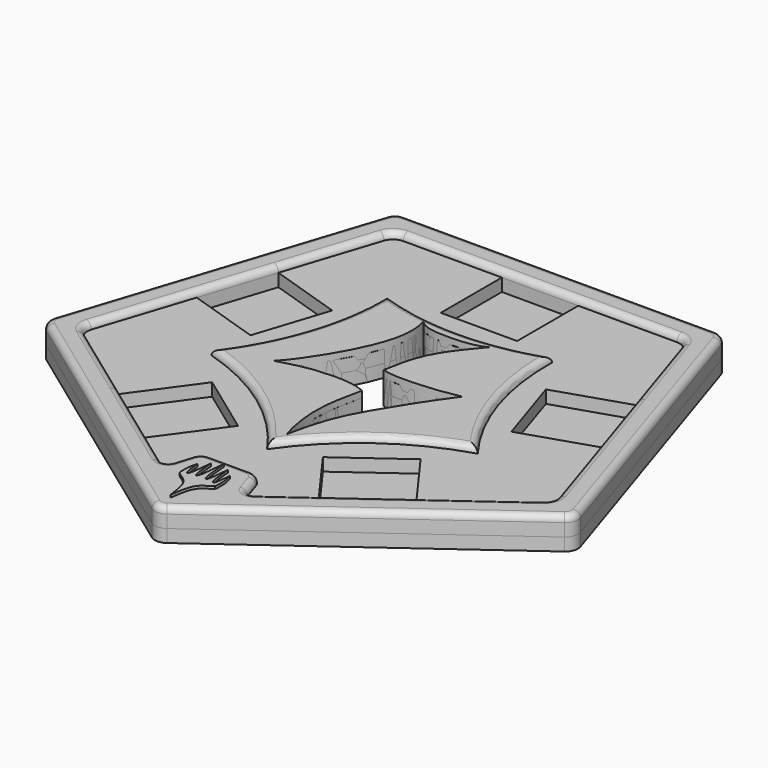
from build123d import *

# Parameters (mm, degrees)
F4_DEPTH      = 2
F5_DEPTH      = 5
F6_DEPTH      = 2
F8_DEPTH      = 5
F9_DEPTH      = 5.001
F10_DEPTH     = 5.4
F11_T2_ANGLE  = 45.9808997244
F11_T4_ANGLE  = 45.9808997244
F11_T6_ANGLE  = 45.9808997244
F11_T8_ANGLE  = 45.9808997244
F11_T10_ANGLE = 45.9808997244
F12_R         = 2
F12_2_R       = 2
F13_R         = 2
F14_R         = 1
F15_R         = 1
F16_R         = 1


# Not quite as in the source:
# - a fillet or chamfer that OpenCascade refuses, or shapes differently, is made with other operations: its cross-section is extruded or revolved along the edge and cut away or added


with BuildPart() as f4:
    # F2 (on Top) → F4 (new body)
    with BuildSketch(Plane.XY):
        Polygon((0, -44), (41.846486717, -13.5967477525), (25.8625511009, 35.5967477525), (-25.8625511009, 35.5967477525), (-41.846486717, -13.5967477525), align=None)
        Polygon((-6.3112691246, -34.4703226653), (-13.7180003831, -29.0890174125), (-23.4262043156, -22.035594385), (-37.1442046986, -12.0688837075), (-31.90439481, 4.0575929247), (-28.1961908775, 15.4702711203), (-22.9563809888, 31.5967477525), (-6, 31.5967477525), (6, 31.5967477525), (22.9563809888, 31.5967477525), (28.1961908775, 15.4702711203), (31.90439481, 4.0575929247), (37.1442046986, -12.0688837075), (23.4262043156, -22.035594385), (13.7180003831, -29.0890174125), (6.3112691246, -34.4703226653), (4.5704734512, -29.0890174125), (-4.6459520236, -29.0890174125), align=None, mode=Mode.SUBTRACT)
        Polygon((-23.4262043156, -22.035594385), (-13.7180003831, -29.0890174125), (-6.3112691246, -34.4703226653), (-4.6459520236, -29.0890174125), (4.5704734512, -29.0890174125), (6.3112691246, -34.4703226653), (13.7180003831, -29.0890174125), (23.4262043156, -22.035594385), (37.1442046986, -12.0688837075), (31.90439481, 4.0575929247), (28.1961908775, 15.4702711203), (22.9563809888, 31.5967477525), (6, 31.5967477525), (-6, 31.5967477525), (-22.9563809888, 31.5967477525), (-28.1961908775, 15.4702711203), (-31.90439481, 4.0575929247), (-37.1442046986, -12.0688837075), align=None)
    extrude(amount=F4_DEPTH)


with BuildPart() as f4b:
    # F0 (on Top) → F4, piece 2 (new body)
    with BuildSketch(Plane.XY):
        Polygon((-16.783512682, 11.7620671878), (-20.4917166145, 0.3493889922), (-31.90439481, 4.0575929247), (-37.1442046986, -12.0688837075), (-23.4262043156, -22.035594385), (-16.3727812881, -12.3273904525), (-6.6645773556, -19.38081348), (-13.7180003831, -29.0890174125), (0, -39.05572809), (13.7180003831, -29.0890174125), (6.6645773556, -19.38081348), (16.3727812881, -12.3273904525), (23.4262043156, -22.035594385), (37.1442046986, -12.0688837075), (31.90439481, 4.0575929247), (20.4917166145, 0.3493889922), (16.783512682, 11.7620671878), (28.1961908775, 15.4702711203), (22.9563809888, 31.5967477525), (6, 31.5967477525), (6, 19.5967477525), (-6, 19.5967477525), (-6, 31.5967477525), (-22.9563809888, 31.5967477525), (-28.1961908775, 15.4702711203), align=None)
        with BuildLine():
            ThreePointArc((0, -22), (-9.1675383126, -12.6180339887), (-20.9232433585, -6.7983738762))
            ThreePointArc((-20.9232433585, -6.7983738762), (-14.833388583, 4.8196601125), (-12.9312755504, 17.7983738762))
            ThreePointArc((-12.9312755504, 17.7983738762), (0, 15.5967477525), (12.9312755504, 17.7983738762))
            ThreePointArc((12.9312755504, 17.7983738762), (14.833388583, 4.8196601125), (20.9232433585, -6.7983738762))
            ThreePointArc((20.9232433585, -6.7983738762), (9.1675383126, -12.6180339887), (0, -22))
        make_face(mode=Mode.SUBTRACT)
        with BuildLine():
            ThreePointArc((-12.9312755504, 17.7983738762), (-14.833388583, 4.8196601125), (-20.9232433585, -6.7983738762))
            ThreePointArc((-20.9232433585, -6.7983738762), (-9.1675383126, -12.6180339887), (0, -22))
            ThreePointArc((0, -22), (9.1675383126, -12.6180339887), (20.9232433585, -6.7983738762))
            ThreePointArc((20.9232433585, -6.7983738762), (14.833388583, 4.8196601125), (12.9312755504, 17.7983738762))
            ThreePointArc((12.9312755504, 17.7983738762), (0, 15.5967477525), (-12.9312755504, 17.7983738762))
        make_face()
    extrude(amount=F4_DEPTH)


with BuildPart() as f5:
    # F2 (on Top) → F5 (new body)
    with BuildSketch(Plane.XY):
        Polygon((0, -44), (41.846486717, -13.5967477525), (25.8625511009, 35.5967477525), (-25.8625511009, 35.5967477525), (-41.846486717, -13.5967477525), align=None)
        Polygon((-6.3112691246, -34.4703226653), (-13.7180003831, -29.0890174125), (-23.4262043156, -22.035594385), (-37.1442046986, -12.0688837075), (-31.90439481, 4.0575929247), (-28.1961908775, 15.4702711203), (-22.9563809888, 31.5967477525), (-6, 31.5967477525), (6, 31.5967477525), (22.9563809888, 31.5967477525), (28.1961908775, 15.4702711203), (31.90439481, 4.0575929247), (37.1442046986, -12.0688837075), (23.4262043156, -22.035594385), (13.7180003831, -29.0890174125), (6.3112691246, -34.4703226653), (4.5704734512, -29.0890174125), (-4.6459520236, -29.0890174125), align=None, mode=Mode.SUBTRACT)
    extrude(amount=F5_DEPTH)

    # F12
    f12_edges = [f5.edges().sort_by_distance(p)[0] for p in [
        (-41.846487, -13.596748, 2.5),
        (0, -44, 2.5),
        (41.846487, -13.596748, 2.5),
        (-25.862551, 35.596748, 2.5),
        (25.862551, 35.596748, 2.5),
        (22.956381, 31.596748, 2.5),
        (-22.956381, 31.596748, 2.5),
        (-37.144205, -12.068884, 2.5),
        (37.144205, -12.068884, 2.5),
    ]]
    fillet(f12_edges, radius=F12_R)

    # F13
    f13_edges = [f5.edges().sort_by_distance(p)[0] for p in [
        (-4.645952, -29.089017, 2.5),
        (4.570473, -29.089017, 2.5),
    ]]
    fillet(f13_edges, radius=F13_R)

    # F14
    f14_edges = [f5.edges().sort_by_distance(p)[0] for p in [
        (-6.311269, -34.470323, 2.5),
        (6.311269, -34.470323, 2.5),
    ]]
    fillet(f14_edges, radius=F14_R)

    # F15
    f15_edges = [f5.edges().sort_by_distance(p)[0] for p in [
        (-25.585037, 35.214782, 5),
    ]]
    fillet(f15_edges, radius=F15_R)

    # F16
    f16_edges = [f5.edges().sort_by_distance(p)[0] for p in [
        (-22.678866, 31.214782, 5),
    ]]
    fillet(f16_edges, radius=F16_R)


with BuildPart() as f6:
    # F6 (new): a face of the model
    f6_faces = [f4b.part.faces().sort_by_distance(p)[0] for p in [
        (0, 0, 2),
    ]]
    extrude(f6_faces, amount=F6_DEPTH)


with BuildPart() as f8:
    # F7 (on Top) → F8 (new body)
    with BuildSketch(Plane.XY):
        with BuildLine():
            ThreePointArc((-12.9312755504, 17.7983738762), (-14.833388583, 4.8196601125), (-20.9232433585, -6.7983738762))
            ThreePointArc((-20.9232433585, -6.7983738762), (-9.1675383126, -12.6180339887), (0, -22))
            ThreePointArc((0, -22), (9.1675383126, -12.6180339887), (20.9232433585, -6.7983738762))
            ThreePointArc((20.9232433585, -6.7983738762), (14.833388583, 4.8196601125), (12.9312755504, 17.7983738762))
            ThreePointArc((12.9312755504, 17.7983738762), (0, 15.5967477525), (-12.9312755504, 17.7983738762))
        make_face()
    extrude(amount=F8_DEPTH)


with BuildPart() as f9_tool:
    # F1 (on Top) → F9 (new body, through all)
    with BuildSketch(Plane.XY):
        with BuildLine():
            add(Edge.make_bspline(
                [(-5.0055538304, 14.9533972144), (-4.0487837978, 13.9171266928), (-1.018710697, 13.4962423882), (3.7661776878, 13.7583203614), (5.5207042024, 14.6353710443)],
                knots=[0, 0, 0, 0, 0.4431624112, 1, 1, 1, 1], degree=3))
            add(Edge.make_bspline(
                [(-12.8237102181, -4.6581095085), (-10.9015761102, -2.6567154814), (-5.9246891757, 4.8908159994), (-4.0491446853, 11.6849951446), (-5.0055538304, 14.9533972144)],
                knots=[0, 0, 0, 0, 0.5143882076, 1, 1, 1, 1], degree=3))
            add(Edge.make_bspline(
                [(0.5711051635, -4.0989685804), (-1.3402187033, -3.1425207853), (-6.6100283409, -3.2325331513), (-9.314772673, -3.6214792635), (-12.8237102181, -4.6581095085)],
                knots=[0, 0, 0, 0, 0.4896183472, 1, 1, 1, 1], degree=3))
            add(Edge.make_bspline(
                [(0.5711051635, -18.9267303795), (-0.0721216688, -16.8167317282), (-1.0198466414, -11.582890578), (-0.06544716, -6.9283478439), (0.5711051635, -4.0989685804)],
                knots=[0, 0, 0, 0, 0.4894776465, 1, 1, 1, 1], degree=3))
            add(Edge.make_bspline(
                [(11.1805992201, 2.3591015488), (8.5564401921, -1.1972968715), (3.7057301296, -8.8437093715), (1.6884206561, -13.4260291234), (0.5711051635, -18.9267303795)],
                knots=[0, 0, 0, 0, 0.5136535404, 1, 1, 1, 1], degree=3))
            add(Edge.make_bspline(
                [(-0.781193783, 1.8798212986), (0.2209486548, 1.5627136075), (3.1716631513, 1.3429362445), (8.0571052822, 1.7147158348), (11.1805992201, 2.3591015488)],
                knots=[0, 0, 0, 0, 0.3994528604, 1, 1, 1, 1], degree=3))
            add(Edge.make_bspline(
                [(5.5207042024, 14.6353710443), (3.7752729912, 12.5626865989), (0.4444851961, 8.5817184971), (-0.4177290348, 4.0256402564), (-0.781193783, 1.8798212986)],
                knots=[0, 0, 0, 0, 0.5211081889, 1, 1, 1, 1], degree=3))
        make_face()
    extrude(amount=F9_DEPTH)


with BuildPart() as f4_1:
    add(f4.part)

    # F9: cut by f9_tool
    add(f9_tool.part, mode=Mode.SUBTRACT)

    # F12#2
    f12_2_edges = [f4_1.edges().sort_by_distance(p)[0] for p in [
        (-41.846487, -13.596748, 1),
        (0, -44, 1),
        (41.846487, -13.596748, 1),
        (-25.862551, 35.596748, 1),
        (25.862551, 35.596748, 1),
    ]]
    fillet(f12_2_edges, radius=F12_2_R)


with BuildPart() as f4b_1:
    add(f4b.part)

    # F9: cut by f9_tool
    add(f9_tool.part, mode=Mode.SUBTRACT)


with BuildPart() as f6_1:
    add(f6.part)

    # F9: cut by f9_tool
    add(f9_tool.part, mode=Mode.SUBTRACT)


with BuildPart() as f8_1:
    add(f8.part)

    # F9: cut by f9_tool
    add(f9_tool.part, mode=Mode.SUBTRACT)

    # F11: fillet of radius 1 on 5 edges, made by hand

    # F11_s1 → F11_t2 (revolve, cut)
    with BuildSketch(Plane(origin=(-20.8061618633, 4.8071339381, 0), x_dir=(0, 0, 1), z_dir=(-0.9743325561, 0.2251134605, 0))):
        with BuildLine():
            ThreePointArc((5, -10.2540254421), (4.7071067812, -10.9611322233), (4, -11.2540254421))
            Line((4, -11.2540254421), (5, -11.2540254421))
            Line((5, -11.2540254421), (5, -10.2540254421))
        make_face()
    revolve(axis=Axis((-32.1363100686, -44.231836169, 5), (0, 0, -1)), revolution_arc=F11_T2_ANGLE, mode=Mode.SUBTRACT)

    # F11_s3 → F11_t4 (revolve, cut)
    with BuildSketch(Plane(origin=(-11.0013136601, -18.3023497381, 0), x_dir=(0, 0, 1), z_dir=(-0.5151809416, -0.8570814416, 0))):
        with BuildLine():
            ThreePointArc((5, -10.2540254421), (4.7071067812, -10.9611322233), (4, -11.2540254421))
            Line((4, -11.2540254421), (5, -11.2540254421))
            Line((5, -11.2540254421), (5, -10.2540254421))
        make_face()
    revolve(axis=Axis((32.1363100686, -44.231836169, 5), (0, 0, -1)), revolution_arc=F11_T4_ANGLE, mode=Mode.SUBTRACT)

    # F11_s5 → F11_t6 (revolve, cut)
    with BuildSketch(Plane(origin=(14.0069761005, -16.1186081503, 0), x_dir=(0, 0, 1), z_dir=(0.6559332239, -0.7548189225, 0))):
        with BuildLine():
            ThreePointArc((4, -11.2540254421), (4.7071067812, -10.9611322233), (5, -10.2540254421))
            Line((5, -10.2540254421), (5, -11.2540254421))
            Line((5, -11.2540254421), (4, -11.2540254421))
        make_face()
    revolve(axis=Axis((51.997641964, 16.8950580318, 5), (0, 0, -1)), revolution_arc=F11_T6_ANGLE, mode=Mode.SUBTRACT)

    # F11_s7 → F11_t8 (revolve, cut)
    with BuildSketch(Plane(origin=(19.6581009698, 8.3405020499, 0), x_dir=(0, 0, 1), z_dir=(0.9205699683, 0.3905776921, 0))):
        with BuildLine():
            ThreePointArc((4, -11.2540254421), (4.7071067812, -10.9611322233), (5, -10.2540254421))
            Line((5, -10.2540254421), (5, -11.2540254421))
            Line((5, -11.2540254421), (4, -11.2540254421))
        make_face()
    revolve(axis=Axis((0, 54.6735562746, 5), (0, 0, -1)), revolution_arc=F11_T8_ANGLE, mode=Mode.SUBTRACT)

    # F11_s9 → F11_t10 (revolve, cut)
    with BuildSketch(Plane(origin=(-1.8576015469, 21.2733219003, 0), x_dir=(0, 0, 1), z_dir=(-0.0869896945, 0.9962092115, 0))):
        with BuildLine():
            ThreePointArc((4, -11.2540254421), (4.7071067812, -10.9611322233), (5, -10.2540254421))
            Line((5, -10.2540254421), (5, -11.2540254421))
            Line((5, -11.2540254421), (4, -11.2540254421))
        make_face()
    revolve(axis=Axis((-51.997641964, 16.8950580318, 5), (0, 0, -1)), revolution_arc=F11_T10_ANGLE, mode=Mode.SUBTRACT)


with BuildPart() as f10:
    # F3 (on Top) → F10 (new body)
    with BuildSketch(Plane.XY):
        with BuildLine():
            add(Edge.make_bspline(
                [(0, -30.4504483938), (0.2669392561, -33.8200293481), (0.5918683268, -35.295922974), (1.0815636488, -34.9679104984), (1.3407623628, -31.3576422632)],
                knots=[0, 0, 0, 0, 0.5276829408, 1, 1, 1, 1], degree=3))
            add(Edge.make_bspline(
                [(0, -30.4504483938), (-0.2669392561, -33.8200293481), (-0.5918683268, -35.295922974), (-1.0815636488, -34.9679104984), (-1.3407623628, -31.3576422632)],
                knots=[0, 0, 0, 0, 0.5276829408, 1, 1, 1, 1], degree=3))
            add(Edge.make_bspline(
                [(-1.3407623628, -31.3576422632), (-1.5614796399, -34.3005402164), (-2.0094542891, -35.7696162636), (-2.3791316307, -34.655806258), (-2.5287040044, -32.4870087206)],
                knots=[0, 0, 0, 0, 0.5441019451, 1, 1, 1, 1], degree=3))
            add(Edge.make_bspline(
                [(-2.5287040044, -32.4870087206), (-2.9020492006, -33.5323778992), (-2.8677394799, -34.4664439392), (-2.9317727527, -35.4883820992), (-2.8033838607, -35.7084795833)],
                knots=[0, 0, 0, 0, 0.5933054686, 1, 1, 1, 1], degree=3))
            add(Edge.make_bspline(
                [(-2.8033838607, -35.7084795833), (-2.4701282382, -36.0972769558), (-0.4448397967, -36.8399446557), (-0.2431228996, -39.4417788186), (0, -40.9665107727)],
                knots=[0, 0, 0, 0, 0.423582582, 1, 1, 1, 1], degree=3))
            add(Edge.make_bspline(
                [(2.8033838607, -35.7084795833), (2.4701282382, -36.0972769558), (0.4448397967, -36.8399446557), (0.2431228996, -39.4417788186), (0, -40.9665107727)],
                knots=[0, 0, 0, 0, 0.423582582, 1, 1, 1, 1], degree=3))
            add(Edge.make_bspline(
                [(2.5287040044, -32.4870087206), (2.9020492006, -33.5323778992), (2.8677394799, -34.4664439392), (2.9317727527, -35.4883820992), (2.8033838607, -35.7084795833)],
                knots=[0, 0, 0, 0, 0.5933054686, 1, 1, 1, 1], degree=3))
            add(Edge.make_bspline(
                [(1.3407623628, -31.3576422632), (1.5614796399, -34.3005402164), (2.0094542891, -35.7696162636), (2.3791316307, -34.655806258), (2.5287040044, -32.4870087206)],
                knots=[0, 0, 0, 0, 0.5441019451, 1, 1, 1, 1], degree=3))
        make_face()
    extrude(amount=F10_DEPTH)


solid = Compound([f5.part, f4_1.part, f4b_1.part, f6_1.part, f8_1.part, f10.part])
